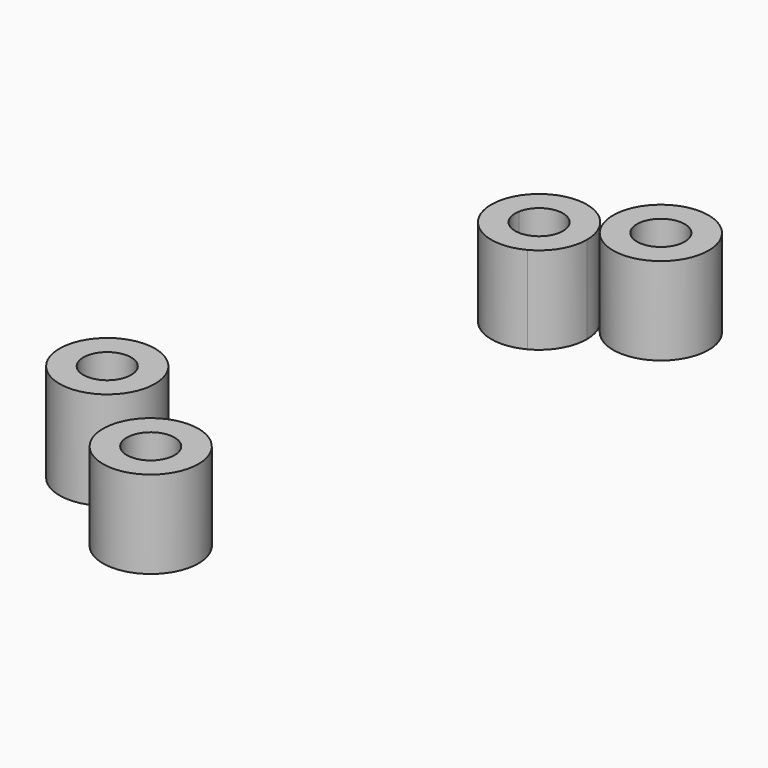
from build123d import *

# Parameters (mm, degrees)
F1_DEPTH = 22
F0_R     = 12
F0_R_2   = 6
F2_DEPTH = 24.7


# Not quite as in the source:
# - a feature names something its author has since deleted; it is built from what else it names


with BuildPart() as f1:
    # F0 (on Top) → F1 (new body)
    with BuildSketch(Plane.XY):
        with BuildLine():
            ThreePointArc((-32.5005938447, 55.2878030792), (-38.2826283024, 56.4801969788), (-40.2442501608, 62.0484790627))
            ThreePointArc((-40.2442501608, 62.0484790627), (-42.8763850896, 63.6632298081), (-45.6252412401, 65.070121459))
            ThreePointArc((-45.6252412401, 65.070121459), (-42.2286871779, 51.9603939576), (-28.7805601487, 50.3637054901))
            ThreePointArc((-28.7805601487, 50.3637054901), (-30.5454719824, 52.897603766), (-32.5005938447, 55.2878030792))
        make_face()
        with BuildLine():
            ThreePointArc((-40.2442501608, 62.0484790627), (-33.8103016262, 66.9768756221), (-28.3365694268, 61))
            ThreePointArc((-28.3365694268, 61), (-29.4880720569, 57.465587283), (-32.5005938447, 55.2878030792))
            ThreePointArc((-32.5005938447, 55.2878030792), (-30.5454719824, 52.897603766), (-28.7805601487, 50.3637054901))
            ThreePointArc((-28.7805601487, 50.3637054901), (-24.0732339227, 54.7819662005), (-22.3365694268, 61))
            ThreePointArc((-22.3365694268, 61), (-32.2706630591, 72.8208303803), (-45.6252412401, 65.070121459))
            ThreePointArc((-45.6252412401, 65.070121459), (-42.8763850896, 63.6632298081), (-40.2442501608, 62.0484790627))
        make_face()
    extrude(amount=F1_DEPTH)


with BuildPart() as f1b:
    # F0 (on Top) → F1, piece 2 (new body)
    with BuildSketch(Plane.XY):
        with Locations((-34.3365694268, -61)):
            Circle(F0_R)
        with Locations((-34.3365694268, -61)):
            Circle(F0_R_2, mode=Mode.SUBTRACT)
    extrude(amount=F1_DEPTH)


with BuildPart() as f1c:
    # F0 (on Top) → F1, piece 3 (new body)
    with BuildSketch(Plane.XY):
        with Locations((-12.8330777054, 72.3710032859)):
            Circle(F0_R)
        with Locations((-12.8330777054, 72.3710032859)):
            Circle(F0_R_2, mode=Mode.SUBTRACT)
    extrude(amount=F1_DEPTH)


with BuildPart() as f2:
    # F0 (on Top) → F2 (new body)
    with BuildSketch(Plane.XY):
        with Locations((-59.0432177121, -43.7738328479)):
            Circle(F0_R)
        with Locations((-59.0432177121, -43.7738328479)):
            Circle(F0_R_2, mode=Mode.SUBTRACT)
    extrude(amount=F2_DEPTH)


solid = Compound([f1.part, f1b.part, f1c.part, f2.part])
